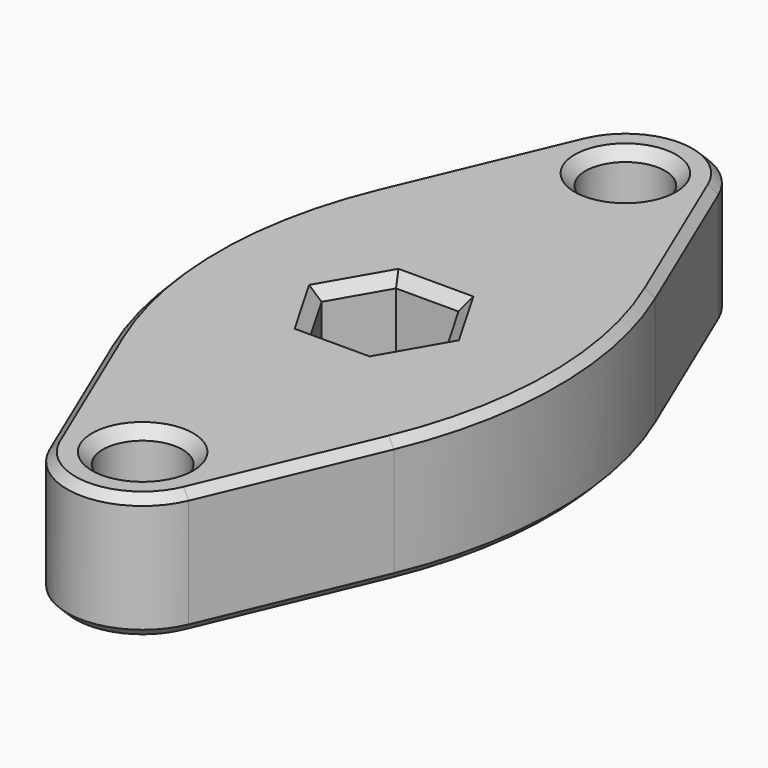
from build123d import *

# Parameters (mm, degrees)
F0_R     = 4.75
F1_DEPTH = 7.5
F2_R     = 50
F3_SIZE  = 1
F4_SCALE = 0.62
F6_DEPTH = 25
F7_SIZE  = 0.8


with BuildPart() as f1:
    # F0 (on Top) → F1 (new body, symmetric)
    with BuildSketch(Plane.XY):
        with BuildLine():
            Line((25, 0), (8.2889389183, 39.5062075821))
            ThreePointArc((8.2889389183, 39.5062075821), (0, 45), (-8.2889389183, 39.5062075821))
            Line((-8.2889389183, 39.5062075821), (-25, 0))
            Line((-25, 0), (-8.2889389183, -39.5062075821))
            ThreePointArc((-8.2889389183, -39.5062075821), (0, -45), (8.2889389183, -39.5062075821))
            Line((8.2889389183, -39.5062075821), (25, 0))
        make_face()
        with Locations((0, -36)):
            Circle(F0_R, mode=Mode.SUBTRACT)
        with Locations((0, 36)):
            Circle(F0_R, mode=Mode.SUBTRACT)
    extrude(amount=F1_DEPTH, both=True)

    # F2
    f2_edges = [f1.edges().sort_by_distance(p)[0] for p in [
        (-25, 0, 0),
        (25, 0, 0),
    ]]
    fillet(f2_edges, radius=F2_R)

    # F3
    f3_edges = [f1.edges().sort_by_distance(p)[0] for p in [
        (0, 45, 7.5),
        (0, 45, -7.5),
        (-12.524692, -29.492569, 7.5),
        (-12.524692, -29.492569, -7.5),
    ]]
    chamfer(f3_edges, length=F3_SIZE)


with BuildPart() as f1_1:
    # F4: moved
    add(f1.part.scale(F4_SCALE))

    # F5 (on face) → F6 (cut)
    with BuildSketch(Plane.XY.offset(4.65)):
        Polygon((-2.3094010768, 4), (-4.6188021535, 0), (-2.3094010768, -4), (2.3094010768, -4), (4.6188021535, 0), (2.3094010768, 4), align=None)
    extrude(amount=-F6_DEPTH, mode=Mode.SUBTRACT)

    # F7
    f7_edges = [f1_1.edges().sort_by_distance(p)[0] for p in [
        (0, -4, 4.65),
        (-3.464102, -2, 4.65),
        (-3.464102, 2, 4.65),
        (0, 4, 4.65),
        (3.464102, 2, 4.65),
        (3.464102, -2, 4.65),
        (0, -4, -4.65),
        (3.464102, -2, -4.65),
        (3.464102, 2, -4.65),
        (0, 4, -4.65),
        (-3.464102, 2, -4.65),
        (-2.945, -22.32, 4.65),
        (-2.945, 22.32, 4.65),
        (-2.945, -22.32, -4.65),
        (-2.945, 22.32, -4.65),
    ]]
    chamfer(f7_edges, length=F7_SIZE)


solid = f1_1.part
